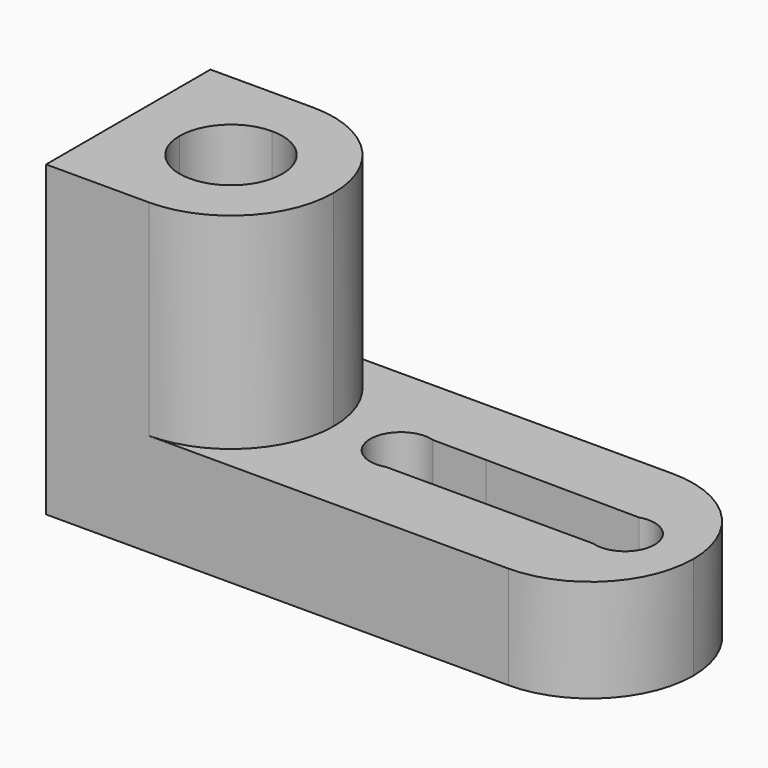
from build123d import *

# Parameters (mm, degrees)
F1_DEPTH = 25.4
F3_DEPTH = 25.4
F5_DEPTH = 25.4
F7_DEPTH = 25.4
F9_DEPTH = 25.4


# Not quite as in the source:
# - a feature names something its author has since deleted; it is built from what else it names


with BuildPart() as f1:
    # F0 (on Front) → F1 (new body)
    with BuildSketch(Plane.XZ):
        Polygon((-5.5358944303, 38.1), (-30.9358944303, 38.1), (-30.9358944303, 0), (38.9141055698, 0), (38.9141055697, 12.7), (-5.5358944303, 12.7), align=None)
    extrude(amount=F1_DEPTH)

    # F2 (on face) → F3 (cut)
    with BuildSketch(Plane.XY.offset(38.1)):
        with BuildLine():
            ThreePointArc((-11.8858944302, -12.7), (-13.7457663697, -8.2098719395), (-18.2358944302, -6.35))
            Line((-18.2358944303, -6.35), (-18.2358944303, -12.7))
            Line((-18.2358944302, -12.7), (-11.8858944302, -12.7))
        make_face()
        with BuildLine():
            Line((-11.8858944302, -12.7), (-18.2358944302, -12.7))
            Line((-18.2358944303, -12.7), (-18.2358944303, -19.05))
            ThreePointArc((-18.2358944302, -19.05), (-13.7457663697, -17.1901280605), (-11.8858944302, -12.7))
        make_face()
        with BuildLine():
            Line((-18.2358944302, -12.7), (-24.5858944303, -12.7))
            ThreePointArc((-24.5858944303, -12.7), (-22.7260224908, -17.1901280605), (-18.2358944302, -19.05))
            Line((-18.2358944303, -19.05), (-18.2358944303, -12.7))
        make_face()
        with BuildLine():
            Line((-18.2358944303, -12.7), (-18.2358944303, -6.35))
            ThreePointArc((-18.2358944302, -6.35), (-22.7260224908, -8.2098719395), (-24.5858944303, -12.7))
            Line((-24.5858944303, -12.7), (-18.2358944302, -12.7))
        make_face()
        with BuildLine():
            Line((-5.5358944303, 0), (-18.2358944303, 0))
            ThreePointArc((-18.2358944303, 0), (-9.2556383092, -3.7197438789), (-5.5358944303, -12.7))
            Line((-5.5358944303, -12.7), (-5.5358944303, 0))
        make_face()
        with BuildLine():
            Line((-5.5358944303, -25.4), (-5.5358944303, -12.7))
            ThreePointArc((-5.5358944303, -12.7), (-9.2556383092, -21.6802561211), (-18.2358944303, -25.4))
            Line((-18.2358944303, -25.4), (-5.5358944303, -25.4))
        make_face()
    extrude(amount=-F3_DEPTH, mode=Mode.SUBTRACT)

    # F4 (on face) → F5 (cut)
    with BuildSketch(Plane.XY.offset(12.7)):
        with BuildLine():
            Line((29.3793692031, -9.1760675128), (10.3391055697, -9.0105000585))
            Line((10.3391055697, -9.0105000585), (10.3391055697, -16.195377335))
            Line((10.3391055697, -16.195377335), (29.3492708089, -16.195377335))
            ThreePointArc((29.3492708089, -16.195377335), (26.7811699001, -12.6746460258), (29.3793692031, -9.1760675128))
        make_face()
        with BuildLine():
            Line((10.3391055697, -16.195377335), (10.3391055697, -9.0105000585))
            Line((10.3391055697, -9.0105000585), (3.7719008779, -8.9533939498))
            ThreePointArc((3.7719008779, -8.9533939498), (5.7024746114, -10.3218470376), (6.442491519, -12.5695466995))
            ThreePointArc((6.442491519, -12.5695466995), (5.6925301995, -14.8306497777), (3.7399555387, -16.195377335))
            Line((3.7399555387, -16.195377335), (10.3391055697, -16.195377335))
        make_face()
        with BuildLine():
            ThreePointArc((34.132825273, -12.6904076897), (32.6422382322, -9.7346534929), (29.3793692031, -9.1760675128))
            Line((29.3793692031, -9.1760675128), (30.4569806904, -9.1854380444))
            Line((30.4569806904, -9.1854380444), (30.4569806904, -16.195377335))
            Line((30.4569806904, -16.195377335), (29.3492708089, -16.195377335))
            ThreePointArc((29.3492708089, -16.195377335), (32.6295441565, -15.6555048856), (34.132825273, -12.6904076897))
        make_face()
        with BuildLine():
            Line((30.4569806904, -9.1854380444), (29.3793692031, -9.1760675128))
            ThreePointArc((29.3793692031, -9.1760675128), (26.7811699001, -12.6746460258), (29.3492708089, -16.195377335))
            Line((29.3492708089, -16.195377335), (30.4569806904, -16.195377335))
            Line((30.4569806904, -16.195377335), (30.4569806904, -9.1854380444))
        make_face()
        with BuildLine():
            ThreePointArc((6.442491519, -12.5695466995), (5.7024746114, -10.3218470376), (3.7719008779, -8.9533939498))
            Line((3.7719008779, -8.9533939498), (2.6589436457, -8.9437160641))
            Line((2.6589436457, -8.9437160641), (2.6589436457, -16.195377335))
            Line((2.6589436457, -16.195377335), (3.7399555387, -16.195377335))
            ThreePointArc((3.7399555387, -16.195377335), (5.6925301995, -14.8306497777), (6.442491519, -12.5695466995))
        make_face()
        with BuildLine():
            Line((2.6589436457, -8.9437160641), (3.7719008779, -8.9533939498))
            ThreePointArc((3.7719008779, -8.9533939498), (-1.1245674179, -12.5528571357), (3.7399555387, -16.195377335))
            Line((3.7399555387, -16.195377335), (2.6589436457, -16.195377335))
            Line((2.6589436457, -16.195377335), (2.6589436457, -8.9437160641))
        make_face()
    extrude(amount=-F5_DEPTH, mode=Mode.SUBTRACT)

    # F6 (on face) → F7 (cut)
    with BuildSketch(Plane.XY.offset(12.7)):
        with BuildLine():
            Line((38.9141055697, -12.7), (38.9141055697, 0))
            Line((38.9141055697, 0), (26.2141055698, 0))
            ThreePointArc((26.2141055698, 0), (35.1943616908, -3.7197438789), (38.9141055697, -12.7))
        make_face()
    extrude(amount=-F7_DEPTH, mode=Mode.SUBTRACT)

    # F8 (on face) → F9 (cut)
    with BuildSketch(Plane.XY.offset(12.7)):
        with BuildLine():
            Line((38.9141055697, -25.4), (38.9141055697, -12.7))
            ThreePointArc((38.9141055697, -12.7), (35.1943616908, -21.6802561211), (26.2141055698, -25.4))
            Line((26.2141055698, -25.4), (38.9141055697, -25.4))
        make_face()
    extrude(amount=-F9_DEPTH, mode=Mode.SUBTRACT)


solid = f1.part
